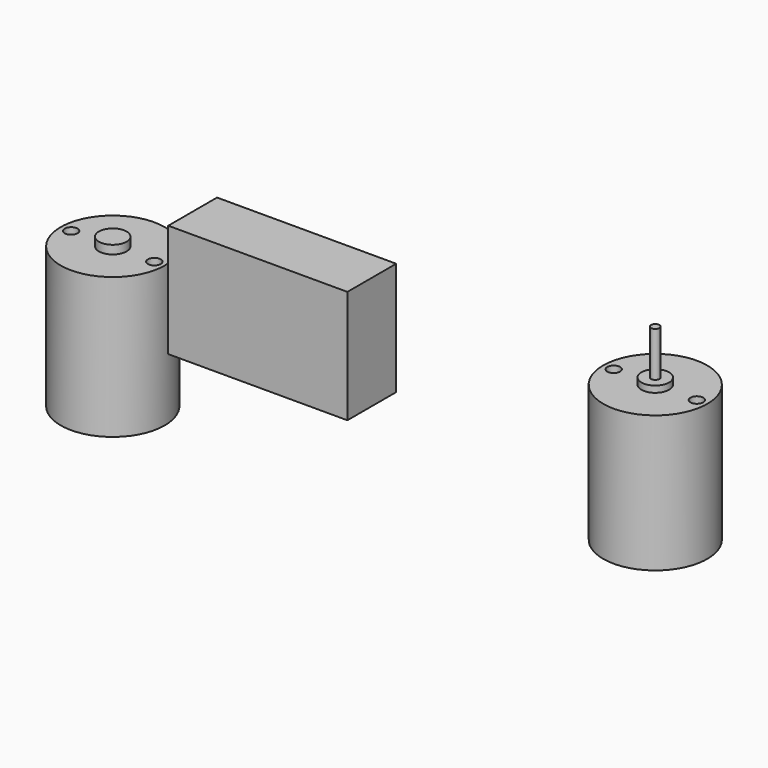
from build123d import *

# Parameters (mm, degrees)
F0_W      = 42
F0_H      = 26.5
F1_DEPTH  = 7.15
F3_R      = 12.2
F3_R_2    = 1.5
F3_R_3    = 3.25
F3_R_4    = 1
F4_DEPTH  = 33
F5_DEPTH  = 2
F7_DEPTH  = 5
F10_DEPTH = 32
F11_DEPTH = 5
F12_DEPTH = 1.5
F13_DEPTH = 12


# Not quite as in the source:
# - the program builds the solid bodies; features that only make, move or delete a surface that nothing else refers to are left out


with BuildPart() as f1:
    # F0 (on Front) → F1 (new body, symmetric)
    with BuildSketch(Plane.XZ):
        Rectangle(F0_W, F0_H)
    extrude(amount=F1_DEPTH, both=True)


with BuildPart() as f4:
    # F3 (on Top) → F4 (new body)
    with BuildSketch(Plane.XY):
        with Locations((-39.7355780005, 0)):
            Circle(F3_R)
        with Locations((-49.4855780005, 0)):
            Circle(F3_R_2, mode=Mode.SUBTRACT)
        with Locations((-39.7355780005, 0)):
            Circle(F3_R_3, mode=Mode.SUBTRACT)
        with Locations((-29.9855780005, 0)):
            Circle(F3_R_2, mode=Mode.SUBTRACT)
        with Locations((-39.7355780005, 0)):
            Circle(F3_R_3)
        with Locations((-39.7355780005, 0)):
            Circle(F3_R_4, mode=Mode.SUBTRACT)
        with Locations((-49.4855780005, 0)):
            Circle(F3_R_2)
        with Locations((-29.9855780005, 0)):
            Circle(F3_R_2)
        with Locations((-39.7355780005, 0)):
            Circle(F3_R_4)
    extrude(amount=-F4_DEPTH)

    # F3 (on Top) → F5 (join)
    with BuildSketch(Plane.XY):
        with Locations((-39.7355780005, 0)):
            Circle(F3_R_3)
        with Locations((-39.7355780005, 0)):
            Circle(F3_R_4, mode=Mode.SUBTRACT)
        with Locations((-39.7355780005, 0)):
            Circle(F3_R_4)
    extrude(amount=F5_DEPTH)

    # F3 (on Top) → F7 (cut)
    with BuildSketch(Plane.XY):
        with Locations((-49.4855780005, 0)):
            Circle(F3_R_2)
        with Locations((-29.9855780005, 0)):
            Circle(F3_R_2)
    extrude(amount=-F7_DEPTH, mode=Mode.SUBTRACT)


with BuildPart() as f10:
    # F9 (on offset) → F10 (new body)
    with BuildSketch(Plane.XY.offset(25)):
        with BuildLine():
            Line((113.3288017511, -18.2856229367), (114.2788017511, -18.2856229367))
            ThreePointArc((114.2788017511, -18.2856229367), (102.0788017511, -6.0856229367), (89.8788017511, -18.2856229367))
            Line((89.8788017511, -18.2856229367), (90.8288017511, -18.2856229367))
            ThreePointArc((90.8288017511, -18.2856229367), (92.3288017511, -16.7856229367), (93.8288017511, -18.2856229367))
            Line((93.8288017511, -18.2856229367), (98.8288017511, -18.2856229367))
            ThreePointArc((98.8288017511, -18.2856229367), (102.0788017511, -15.0356229367), (105.3288017511, -18.2856229367))
            Line((105.3288017511, -18.2856229367), (110.3288017511, -18.2856229367))
            ThreePointArc((110.3288017511, -18.2856229367), (111.8288017511, -16.7856229367), (113.3288017511, -18.2856229367))
        make_face()
        with BuildLine():
            ThreePointArc((89.8788017511, -18.2856229367), (102.0788017511, -30.4856229367), (114.2788017511, -18.2856229367))
            Line((114.2788017511, -18.2856229367), (113.3288017511, -18.2856229367))
            ThreePointArc((113.3288017511, -18.2856229367), (111.8288017511, -19.7856229367), (110.3288017511, -18.2856229367))
            Line((110.3288017511, -18.2856229367), (105.3288017511, -18.2856229367))
            ThreePointArc((105.3288017511, -18.2856229367), (102.0788017511, -21.5356229367), (98.8288017511, -18.2856229367))
            Line((98.8288017511, -18.2856229367), (93.8288017511, -18.2856229367))
            ThreePointArc((93.8288017511, -18.2856229367), (92.3288017511, -19.7856229367), (90.8288017511, -18.2856229367))
            Line((90.8288017511, -18.2856229367), (89.8788017511, -18.2856229367))
        make_face()
        with BuildLine():
            Line((110.3288017511, -18.2856229367), (113.3288017511, -18.2856229367))
            ThreePointArc((113.3288017511, -18.2856229367), (111.8288017511, -16.7856229367), (110.3288017511, -18.2856229367))
        make_face()
        with BuildLine():
            ThreePointArc((110.3288017511, -18.2856229367), (111.8288017511, -19.7856229367), (113.3288017511, -18.2856229367))
            Line((113.3288017511, -18.2856229367), (110.3288017511, -18.2856229367))
        make_face()
        with BuildLine():
            Line((103.0788017511, -18.2856229367), (105.3288017511, -18.2856229367))
            ThreePointArc((105.3288017511, -18.2856229367), (102.0788017511, -15.0356229367), (98.8288017511, -18.2856229367))
            Line((98.8288017511, -18.2856229367), (101.0788017511, -18.2856229367))
            ThreePointArc((101.0788017511, -18.2856229367), (102.0788017511, -17.2856229367), (103.0788017511, -18.2856229367))
        make_face()
        with BuildLine():
            ThreePointArc((98.8288017511, -18.2856229367), (102.0788017511, -21.5356229367), (105.3288017511, -18.2856229367))
            Line((105.3288017511, -18.2856229367), (103.0788017511, -18.2856229367))
            ThreePointArc((103.0788017511, -18.2856229367), (102.0788017511, -19.2856229367), (101.0788017511, -18.2856229367))
            Line((101.0788017511, -18.2856229367), (98.8288017511, -18.2856229367))
        make_face()
        with BuildLine():
            Line((101.0788017511, -18.2856229367), (103.0788017511, -18.2856229367))
            ThreePointArc((103.0788017511, -18.2856229367), (102.0788017511, -17.2856229367), (101.0788017511, -18.2856229367))
        make_face()
        with BuildLine():
            ThreePointArc((101.0788017511, -18.2856229367), (102.0788017511, -19.2856229367), (103.0788017511, -18.2856229367))
            Line((103.0788017511, -18.2856229367), (101.0788017511, -18.2856229367))
        make_face()
        with BuildLine():
            ThreePointArc((93.8288017511, -18.2856229367), (92.3288017511, -16.7856229367), (90.8288017511, -18.2856229367))
            Line((90.8288017511, -18.2856229367), (93.8288017511, -18.2856229367))
        make_face()
        with BuildLine():
            Line((93.8288017511, -18.2856229367), (90.8288017511, -18.2856229367))
            ThreePointArc((90.8288017511, -18.2856229367), (92.3288017511, -19.7856229367), (93.8288017511, -18.2856229367))
        make_face()
    extrude(amount=-F10_DEPTH)

    # F9 (on offset) → F11 (cut)
    with BuildSketch(Plane.XY.offset(25)):
        with BuildLine():
            ThreePointArc((93.8288017511, -18.2856229367), (92.3288017511, -16.7856229367), (90.8288017511, -18.2856229367))
            Line((90.8288017511, -18.2856229367), (93.8288017511, -18.2856229367))
        make_face()
        with BuildLine():
            Line((93.8288017511, -18.2856229367), (90.8288017511, -18.2856229367))
            ThreePointArc((90.8288017511, -18.2856229367), (92.3288017511, -19.7856229367), (93.8288017511, -18.2856229367))
        make_face()
        with BuildLine():
            Line((110.3288017511, -18.2856229367), (113.3288017511, -18.2856229367))
            ThreePointArc((113.3288017511, -18.2856229367), (111.8288017511, -16.7856229367), (110.3288017511, -18.2856229367))
        make_face()
        with BuildLine():
            ThreePointArc((110.3288017511, -18.2856229367), (111.8288017511, -19.7856229367), (113.3288017511, -18.2856229367))
            Line((113.3288017511, -18.2856229367), (110.3288017511, -18.2856229367))
        make_face()
    extrude(amount=-F11_DEPTH, mode=Mode.SUBTRACT)

    # F9 (on offset) → F12 (join)
    with BuildSketch(Plane.XY.offset(25)):
        with BuildLine():
            Line((103.0788017511, -18.2856229367), (105.3288017511, -18.2856229367))
            ThreePointArc((105.3288017511, -18.2856229367), (102.0788017511, -15.0356229367), (98.8288017511, -18.2856229367))
            Line((98.8288017511, -18.2856229367), (101.0788017511, -18.2856229367))
            ThreePointArc((101.0788017511, -18.2856229367), (102.0788017511, -17.2856229367), (103.0788017511, -18.2856229367))
        make_face()
        with BuildLine():
            ThreePointArc((98.8288017511, -18.2856229367), (102.0788017511, -21.5356229367), (105.3288017511, -18.2856229367))
            Line((105.3288017511, -18.2856229367), (103.0788017511, -18.2856229367))
            ThreePointArc((103.0788017511, -18.2856229367), (102.0788017511, -19.2856229367), (101.0788017511, -18.2856229367))
            Line((101.0788017511, -18.2856229367), (98.8288017511, -18.2856229367))
        make_face()
    extrude(amount=F12_DEPTH)

    # F9 (on offset) → F13 (join)
    with BuildSketch(Plane.XY.offset(25)):
        with BuildLine():
            Line((101.0788017511, -18.2856229367), (103.0788017511, -18.2856229367))
            ThreePointArc((103.0788017511, -18.2856229367), (102.0788017511, -17.2856229367), (101.0788017511, -18.2856229367))
        make_face()
        with BuildLine():
            ThreePointArc((101.0788017511, -18.2856229367), (102.0788017511, -19.2856229367), (103.0788017511, -18.2856229367))
            Line((103.0788017511, -18.2856229367), (101.0788017511, -18.2856229367))
        make_face()
    extrude(amount=F13_DEPTH)


solid = Compound([f1.part, f4.part, f10.part])
